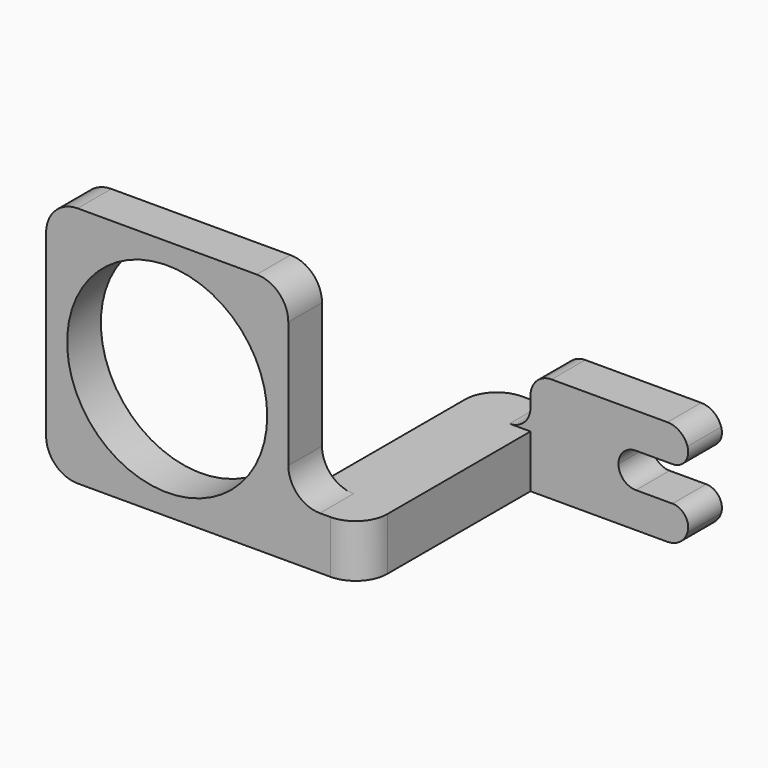
from build123d import *

# Parameters (mm, degrees)
F1_DEPTH  = 5
F0_W      = 23
F0_H      = 4
F2_DEPTH  = 23
F4_R      = 3
F3_R      = 9.5
F5_DEPTH  = 25
F0_W_2    = 15
F6_DEPTH  = 10
F7_R      = 2
F9_DEPTH  = 25
F10_DEPTH = 25
F11_R     = 1.5


with BuildPart() as f1:
    # F0 (on Top) → F1 (new body)
    with BuildSketch(Plane.XY):
        Polygon((-15.8038523793, -12.5927883387), (-15.8038523793, -8.5927883387), (-22.8038523793, -8.5927883387), (-22.8038523793, -28.5927883387), (-22.8038523793, -32.5927883387), (-15.8038523793, -32.5927883387), align=None)
    extrude(amount=F1_DEPTH)

    # F0 (on Top) → F2 (join)
    with BuildSketch(Plane.XY):
        with Locations((-34.3038523793, -30.5927883387)):
            Rectangle(F0_W, F0_H)
    extrude(amount=F2_DEPTH)

    # F4
    f4_edges = [f1.edges().sort_by_distance(p)[0] for p in [
        (-22.803852, -30.592788, 5),
        (-22.803852, -30.592788, 23),
        (-45.803852, -30.592788, 23),
        (-45.803852, -30.592788, 0),
        (-22.803852, -8.592788, 2.5),
        (-15.803852, -32.592788, 2.5),
    ]]
    fillet(f4_edges, radius=F4_R)

    # F3 (on face) → F5 (cut)
    with BuildSketch(Plane.XZ.offset(32.5927883387)):
        with Locations((-34.3038523793, 11.5)):
            Circle(F3_R)
    extrude(amount=-F5_DEPTH, mode=Mode.SUBTRACT)

    # F0 (on Top) → F6 (join)
    with BuildSketch(Plane.XY):
        with Locations((-8.3038523793, -10.5927883387)):
            Rectangle(F0_W_2, F0_H)
    extrude(amount=F6_DEPTH)

    # F7
    f7_edges = [f1.edges().sort_by_distance(p)[0] for p in [
        (-15.803852, -10.592788, 5),
        (-15.803852, -10.592788, 10),
        (-0.803852, -10.592788, 10),
        (-0.803852, -10.592788, 0),
    ]]
    fillet(f7_edges, radius=F7_R)

    # F8 (on face) → F9 (cut)
    with BuildSketch(Plane(origin=(0, -8.5927883387, 0), x_dir=(-1, 0, 0), z_dir=(0, 1, 0))):
        with BuildLine():
            ThreePointArc((5.7965948978, 3.350015961), (6.9680098333, 3.8307107192), (7.4538523793, 5))
            ThreePointArc((7.4538523793, 5), (6.9705785683, 6.166726189), (5.8038523793, 6.65))
            ThreePointArc((5.8038523793, 6.65), (4.1538563696, 5.0036287496), (5.7965948978, 3.350015961))
        make_face()
    extrude(amount=-F9_DEPTH, mode=Mode.SUBTRACT)

    # F8 (on face) → F10 (cut)
    with BuildSketch(Plane(origin=(0, -8.5927883387, 0), x_dir=(-1, 0, 0), z_dir=(0, 1, 0))):
        with BuildLine():
            ThreePointArc((5.7965948978, 3.350015961), (4.1538563696, 5.0036287496), (5.8038523793, 6.65))
            Line((5.8038523793, 6.65), (0.8038523793, 6.65))
            Line((0.8038523793, 6.65), (0.8038523793, 3.350015961))
            Line((0.8038523793, 3.350015961), (5.7965948978, 3.350015961))
        make_face()
    extrude(amount=-F10_DEPTH, mode=Mode.SUBTRACT)

    # F11
    f11_edges = [f1.edges().sort_by_distance(p)[0] for p in [
        (-0.803852, -10.592788, 3.350016),
        (-0.803852, -10.592788, 6.65),
    ]]
    fillet(f11_edges, radius=F11_R)


solid = f1.part
